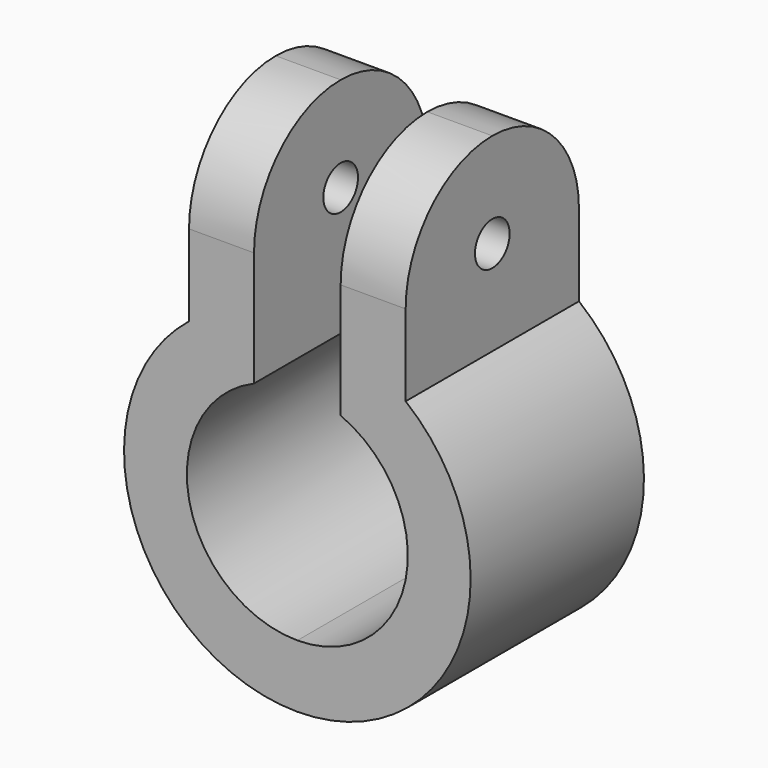
from build123d import *

# Parameters (mm, degrees)
F1_DEPTH = 5
F2_R     = 1
F3_DEPTH = 25
F4_R     = 4.99999


# Not quite as in the source:
# - a fillet or chamfer is up to 0.001 mm smaller than in the source, because OpenCascade refuses the exact size
# - a feature names something its author has since deleted; it is built from what else it names


with BuildPart() as f1:
    # F0 (on Front) → F1 (new body, symmetric)
    with BuildSketch(Plane.XZ):
        with BuildLine():
            ThreePointArc((2, 4.6914816423), (4.9968268119, -1.0206477415), (0, -5.1))
            Line((0, -5.1), (0, -8))
            ThreePointArc((0, -8), (7.5485092564, -2.6495297708), (5, 6.2449979984))
            ThreePointArc((5, 6.2449979984), (3.5795567819, 7.1544932207), (2, 7.7459666924))
            Line((2, 7.7459666924), (2, 4.6914816423))
        make_face()
        with BuildLine():
            Line((2, 15), (2, 7.7459666924))
            ThreePointArc((2, 7.7459666924), (3.5795567819, 7.1544932207), (5, 6.2449979984))
            Line((5, 6.2449979984), (5, 15))
            Line((5, 15), (2, 15))
        make_face()
    extrude(amount=F1_DEPTH, both=True)

    # F2 (on face) → F3 (cut)
    with BuildSketch(Plane.YZ.offset(5)):
        with Locations((0, 10.6224989992)):
            Circle(F2_R)
    extrude(amount=-F3_DEPTH, mode=Mode.SUBTRACT)

    # F4 (radius 5 in the source; OpenCascade refuses exactly that, so slightly less here)
    f4_edges = [f1.edges().sort_by_distance(p)[0] for p in [
        (3.5, -5, 15),
        (3.5, 5, 15),
    ]]
    fillet(f4_edges, radius=F4_R)

    # F5: F1 across plane


with BuildPart() as f1_1:
    add(f1.part)
    add(f1.part.mirror(Plane.YZ))


solid = f1_1.part
